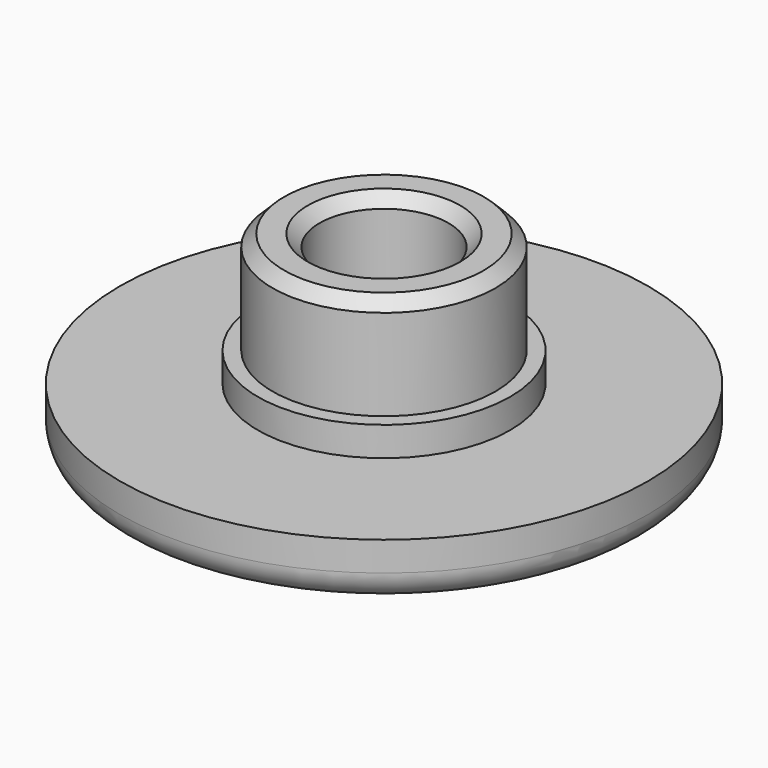
from build123d import *

# Parameters (mm, degrees)
F0_R     = 9
F0_R_2   = 4.3
F1_DEPTH = 2
F0_R_3   = 2.2
F0_R_4   = 3.8
F2_DEPTH = 3
F3_DEPTH = 6.5
F4_R     = 1
F5_SIZE  = 0.4


with BuildPart() as f1:
    # F0 (on Top) → F1 (new body)
    with BuildSketch(Plane.XY):
        Circle(F0_R)
        Circle(F0_R_2, mode=Mode.SUBTRACT)
    extrude(amount=F1_DEPTH)

    # F0 (on Top) → F2 (join)
    with BuildSketch(Plane.XY):
        Circle(F0_R_2)
        Circle(F0_R_4, mode=Mode.SUBTRACT)
    extrude(amount=F2_DEPTH)

    # F0 (on Top) → F3 (join)
    with BuildSketch(Plane.XY):
        Circle(F0_R_4)
        Circle(F0_R_3, mode=Mode.SUBTRACT)
    extrude(amount=F3_DEPTH)

    # F4
    f4_edges = [f1.edges().sort_by_distance(p)[0] for p in [
        (-9, 0, 0),
    ]]
    fillet(f4_edges, radius=F4_R)

    # F5
    f5_edges = [f1.edges().sort_by_distance(p)[0] for p in [
        (-3.8, 0, 6.5),
        (-2.2, 0, 6.5),
    ]]
    chamfer(f5_edges, length=F5_SIZE)


with BuildPart() as f1b:
    # F0 (on Top) → F1, piece 2 (new body)
    with BuildSketch(Plane.XY):
        Circle(F0_R_3)
    extrude(amount=F1_DEPTH)


solid = Compound([f1.part, f1b.part])
